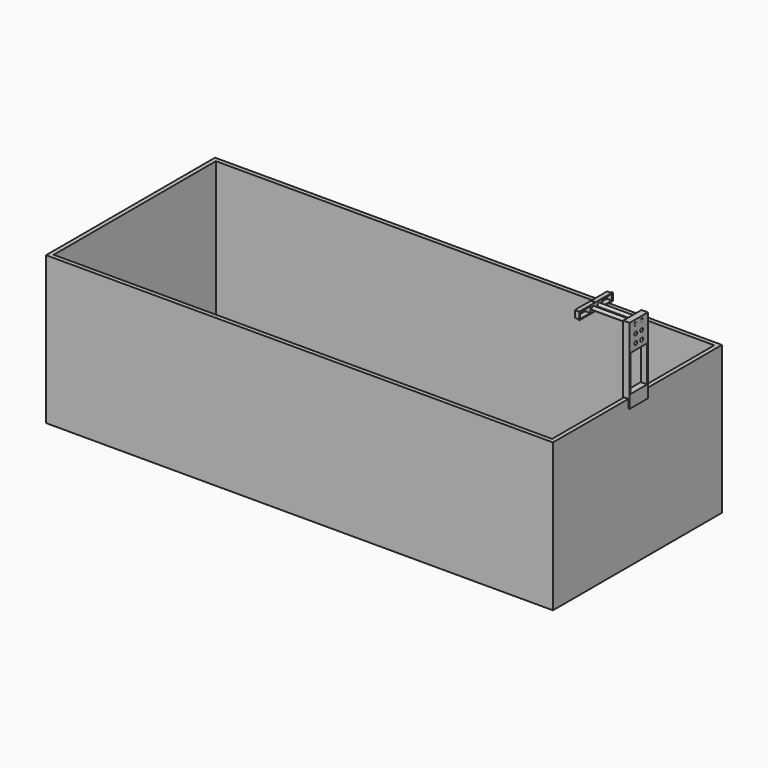
from build123d import *

# Parameters (mm, degrees)
F0_W          = 1.5
F0_H          = 1
F0_H_2        = 16
F0_R          = 4.25
F0_W_2        = 30
F0_H_3        = 14
F1_DEPTH      = 2
F2_DEPTH      = 10
F2_DEPTH_BACK = 2
F5_W          = 1200
F5_H          = 500
F5_W_2        = 1180
F5_H_2        = 480
F6_DEPTH      = 350
F8_W          = 10
F8_H          = 2
F8_W_2        = 1
F8_H_2        = 50
F9_DEPTH      = 10
F10_DEPTH     = 20
F11_R         = 4.25
F12_DEPTH     = 15
F13_W         = 110
F13_H         = 4


# Not quite as in the source:
# - a feature names something its author has since deleted; it is built from what else it names
# - the program builds the solid bodies; features that only make, move or delete a surface that nothing else refers to are left out


with BuildPart() as f1:
    # F0 (on Right) → F1 (new body)
    with BuildSketch(Plane.YZ):
        Polygon((-0.75, 9), (-49.5, 9), (-49.5, -9), (-0.75, -9), (-0.75, -8), (-13, -8), (-16, -8), (-48, -8), (-48, 8), (-16, 8), (-13, 8), (-0.75, 8), align=None)
        with Locations((0, 8.5)):
            Rectangle(F0_W, F0_H)
        Polygon((49.5, 9), (0.75, 9), (0.75, 8), (13, 8), (16, 8), (48, 8), (48, -8), (16, -8), (13, -8), (0.75, -8), (0.75, -9), (49.5, -9), align=None)
        with Locations((0, -8.5)):
            Rectangle(F0_W, F0_H)
        Rectangle(F0_W, F0_H_2)
        Polygon((13, 8), (0.75, 8), (0.75, -8), (13, -8), (16, -8), (48, -8), (48, 8), (16, 8), align=None)
        with Locations((8.75, 0)):
            Circle(F0_R, mode=Mode.SUBTRACT)
        with Locations((32, 0)):
            Rectangle(F0_W_2, F0_H_3, mode=Mode.SUBTRACT)
    extrude(amount=F1_DEPTH)

    # F0 (on Right) → F2 (join, two sides)
    with BuildSketch(Plane.YZ) as f2_sk:
        Polygon((-0.75, -8), (-0.75, 8), (-13, 8), (-16, 8), (-48, 8), (-48, -8), (-16, -8), (-13, -8), align=None)
        with Locations((-32, 0)):
            Rectangle(F0_W_2, F0_H_3, mode=Mode.SUBTRACT)
        with Locations((-8.75, 0)):
            Circle(F0_R, mode=Mode.SUBTRACT)
        Polygon((13, 8), (0.75, 8), (0.75, -8), (13, -8), (16, -8), (48, -8), (48, 8), (16, 8), align=None)
        with Locations((8.75, 0)):
            Circle(F0_R, mode=Mode.SUBTRACT)
        with Locations((32, 0)):
            Rectangle(F0_W_2, F0_H_3, mode=Mode.SUBTRACT)
    extrude(amount=-F2_DEPTH)
    extrude(f2_sk.sketch, amount=F2_DEPTH_BACK)


with BuildPart() as f6:
    # F5 (on offset) → F6 (new body)
    with BuildSketch(Plane.XY.offset(-500)):
        with Locations((-500, 0)):
            Rectangle(F5_W, F5_H)
        with Locations((-500, 0)):
            Rectangle(F5_W_2, F5_H_2, mode=Mode.SUBTRACT)
    extrude(amount=F6_DEPTH)


with BuildPart() as f9:
    # F8 (on face) → F9 (new body)
    with BuildSketch(Plane.XY.offset(-150)):
        Polygon((101, 27), (101, 25), (101, -25), (101, -27), (103, -27), (103, 27), align=None)
        Polygon((90, -25), (90, 25), (90, 27), (88, 27), (88, -27), (90, -27), align=None)
        with Locations((95, 26)):
            Rectangle(F8_W, F8_H)
        with Locations((100.5, 26)):
            Rectangle(F8_W_2, F8_H)
        with Locations((100.5, -26)):
            Rectangle(F8_W_2, F8_H)
        with Locations((95, -26)):
            Rectangle(F8_W, F8_H)
        with Locations((100.5, 0)):
            Rectangle(F8_W_2, F8_H_2)
        with Locations((95, 0)):
            Rectangle(F8_W, F8_H_2)
    extrude(amount=F9_DEPTH)

    # F8 (on face) → F10 (join)
    with BuildSketch(Plane.XY.offset(-150)):
        Polygon((90, -25), (90, 25), (90, 27), (88, 27), (88, -27), (90, -27), align=None)
        Polygon((101, 27), (101, 25), (101, -25), (101, -27), (103, -27), (103, 27), align=None)
    extrude(amount=-F10_DEPTH)

    # F11 (on face) → F12 (join)
    with BuildSketch(Plane.YZ.offset(103)):
        Polygon((-25, -140), (-27, -140), (-27, -150), (27, -150), (27, -140), (25, -140), align=None)
        Polygon((-27, 9.5), (-27, -140), (-25, -140), (-25, -54.25), (25, -54.25), (25, -140), (27, -140), (27, 9.5), align=None)
        with Locations((-8.75, -40)):
            Circle(F11_R, mode=Mode.SUBTRACT)
        with Locations((-8.75, -20)):
            Circle(F11_R, mode=Mode.SUBTRACT)
        with Locations((-8.75, 0)):
            Circle(F11_R, mode=Mode.SUBTRACT)
        with Locations((8.75, -40)):
            Circle(F11_R, mode=Mode.SUBTRACT)
        with Locations((8.75, -20)):
            Circle(F11_R, mode=Mode.SUBTRACT)
        with Locations((8.75, 0)):
            Circle(F11_R, mode=Mode.SUBTRACT)
    extrude(amount=-F12_DEPTH)


with BuildPart() as f14:
    # F13 (on Top) → F14 (revolve)
    with BuildSketch(Plane.XY):
        with Locations((48, -6.5)):
            Rectangle(F13_W, F13_H)
    revolve(axis=Axis((48, -8.5, 0), (1, 0, 0)))


with BuildPart() as f15:
    # F13 (on Top) → F15 (revolve)
    with BuildSketch(Plane.XY):
        with Locations((48, 6.5)):
            Rectangle(F13_W, F13_H)
    revolve(axis=Axis((48, 8.5, 0), (1, 0, 0)))


solid = Compound([f1.part, f6.part, f9.part, f14.part, f15.part])
